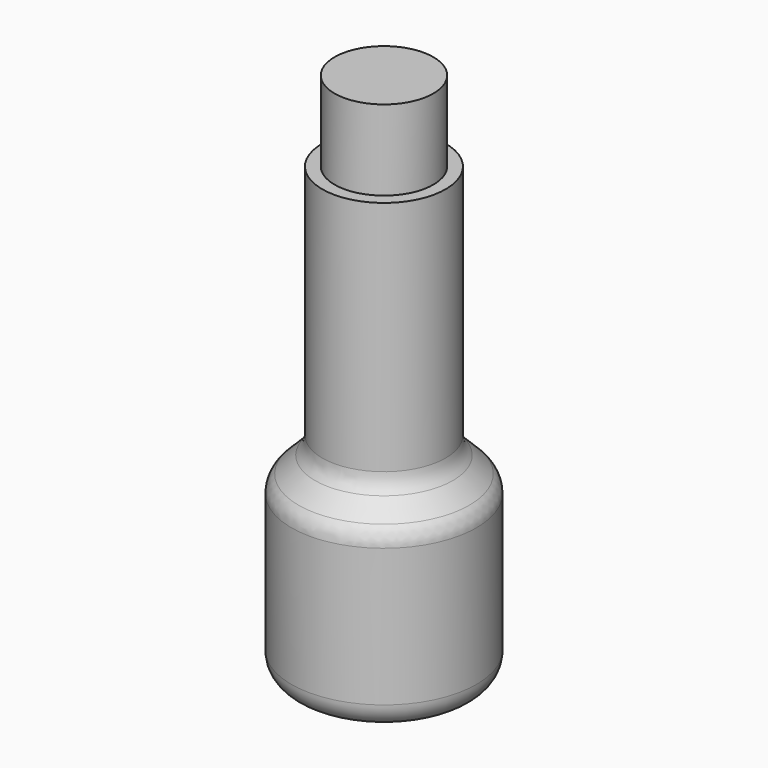
from build123d import *

# Parameters (mm, degrees)
F2_R         = 2
F3_TEXT_SIZE = 10.4166666667
F4_DEPTH     = 2


# Not quite as in the source:
# - Text() gives the source's letters only with a copy of the font that has no kerning and outlines rounded to 1/6400 em; it was checked with that copy


with BuildPart() as f1:
    # F0 (on Right) → F1 (revolve)
    with BuildSketch(Plane.YZ):
        Polygon((-7.5, 0), (0, 0), (0, 43), (-4, 43), (-4, 36.5), (-5, 36.5), (-5, 16.5), (-7.5, 14), align=None)
    revolve(axis=Axis((0, 0, 21.5), (0, 0, -1)))

    # F2
    f2_edges = [f1.edges().sort_by_distance(p)[0] for p in [
        (0, 7.5, 0),
        (0, 7.5, 14),
        (0, 5, 16.5),
    ]]
    fillet(f2_edges, radius=F2_R)

    # F3 (on face) → F4 (cut)
    with BuildSketch(Plane(origin=(0, 0, 0), x_dir=(1, 0, 0), z_dir=(0, 0, -1))):
        with Locations((-3.5578223922, -3.7133955723)):
            Text('R', F3_TEXT_SIZE, font='Arimo', font_style=FontStyle.BOLD, text_align=(TextAlign.LEFT, TextAlign.BOTTOM))
    extrude(amount=-F4_DEPTH, mode=Mode.SUBTRACT)


solid = f1.part
